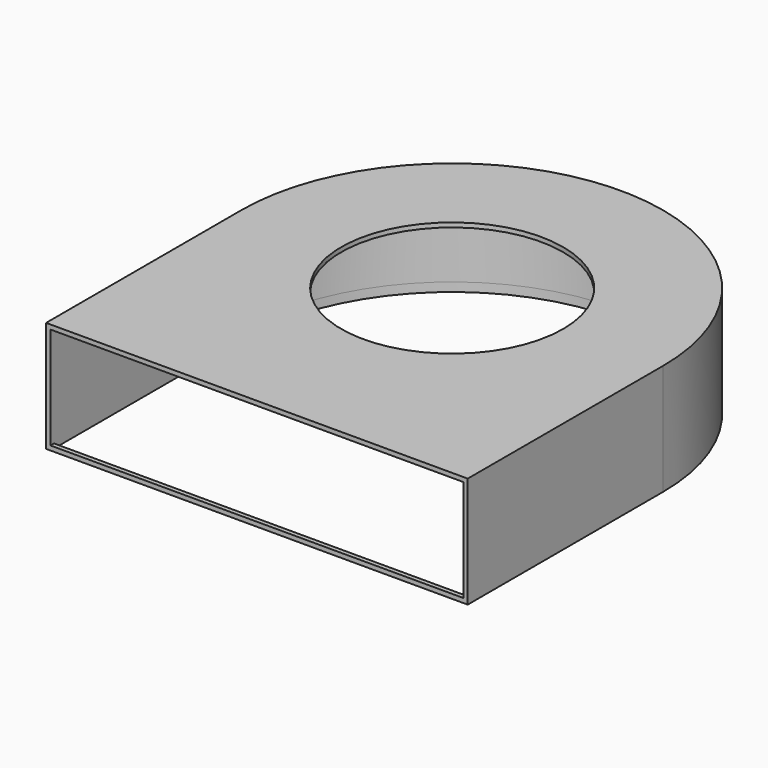
from build123d import *

# Parameters (mm, degrees)
F1_DEPTH = 25
F2_T     = -1
F3_R     = 25
F4_DEPTH = 25.001
F5_R     = 25
F6_DEPTH = 2


# Not quite as in the source:
# - after a boolean that leaves OpenCascade's solid faulty, fix() repairs it


with BuildPart() as f1:
    # F0 (on Top) → F1 (new body)
    with BuildSketch(Plane.XY):
        with BuildLine():
            ThreePointArc((-47.5, 0), (0, -47.5), (47.5, 0))
            ThreePointArc((47.5, 0), (0, 47.5), (-47.5, 0))
        make_face()
        with BuildLine():
            Line((47.5, -55), (47.5, 0))
            ThreePointArc((47.5, 0), (0, -47.5), (-47.5, 0))
            Line((-47.5, 0), (-47.5, -55))
            Line((-47.5, -55), (47.5, -55))
        make_face()
    extrude(amount=F1_DEPTH)

    # F2
    f2_openings = [f1.faces().sort_by_distance(p)[0] for p in [
        (0, -55, 12.5),
    ]]
    offset(amount=F2_T, openings=f2_openings)

    # F3 (on face) → F4 (cut, through all)
    with BuildSketch(Plane.XY.offset(25)):
        Circle(F3_R)
    extrude(amount=-F4_DEPTH, mode=Mode.SUBTRACT)

    # F5 (on face) → F6 (cut)
    with BuildSketch(Plane(origin=(0, 0, 0), x_dir=(1, 0, 0), z_dir=(0, 0, -1))):
        with BuildLine():
            Line((-46.5, 54), (-46.5, 0))
            ThreePointArc((-46.5, 0), (0, -46.5), (46.5, 0))
            Line((46.5, 0), (46.5, 54))
            Line((46.5, 54), (-46.5, 54))
        make_face()
        Circle(F5_R, mode=Mode.SUBTRACT)
        with BuildLine():
            Line((-46.5, 54), (-46.5, 0))
            ThreePointArc((-46.5, 0), (0, -46.5), (46.5, 0))
            Line((46.5, 0), (46.5, 54))
            Line((46.5, 54), (-46.5, 54))
        make_face()
    extrude(amount=-F6_DEPTH, mode=Mode.SUBTRACT)

    add(f1.part.fix(), mode=Mode.REPLACE)


solid = f1.part
